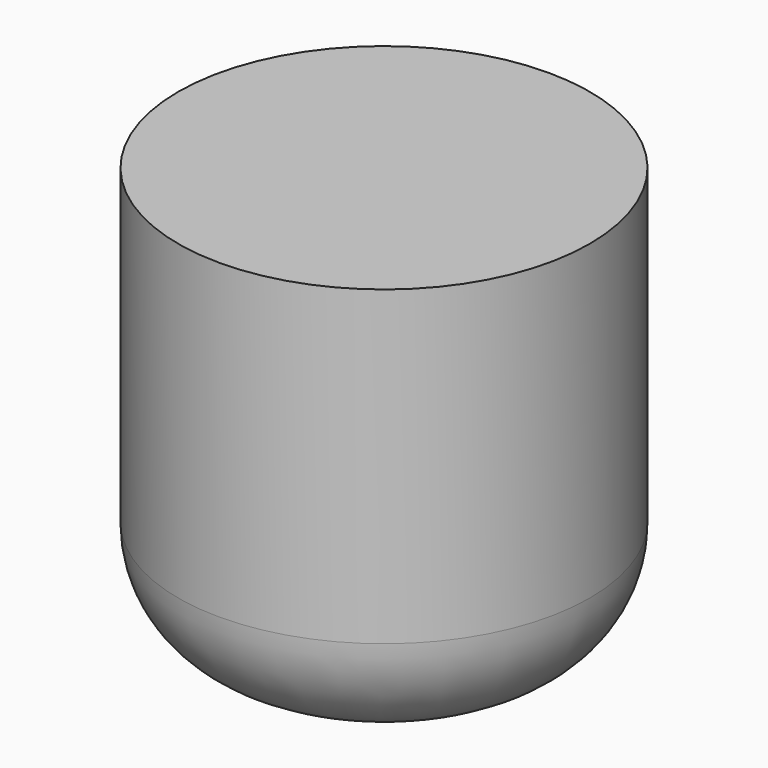
from build123d import *

# Parameters (mm, degrees)
F0_R     = 9.2183658135
F1_DEPTH = 19.05
F5_R     = 5.08


# Not quite as in the source:
# - the program builds the solid bodies; features that only make, move or delete a surface that nothing else refers to are left out


with BuildPart() as f1:
    # F0 (on Top) → F1 (new body)
    with BuildSketch(Plane.XY):
        Circle(F0_R)
    extrude(amount=F1_DEPTH)

    # F5
    f5_edges = [f1.edges().sort_by_distance(p)[0] for p in [
        (-9.218366, 0, 0),
    ]]
    fillet(f5_edges, radius=F5_R)


solid = f1.part
